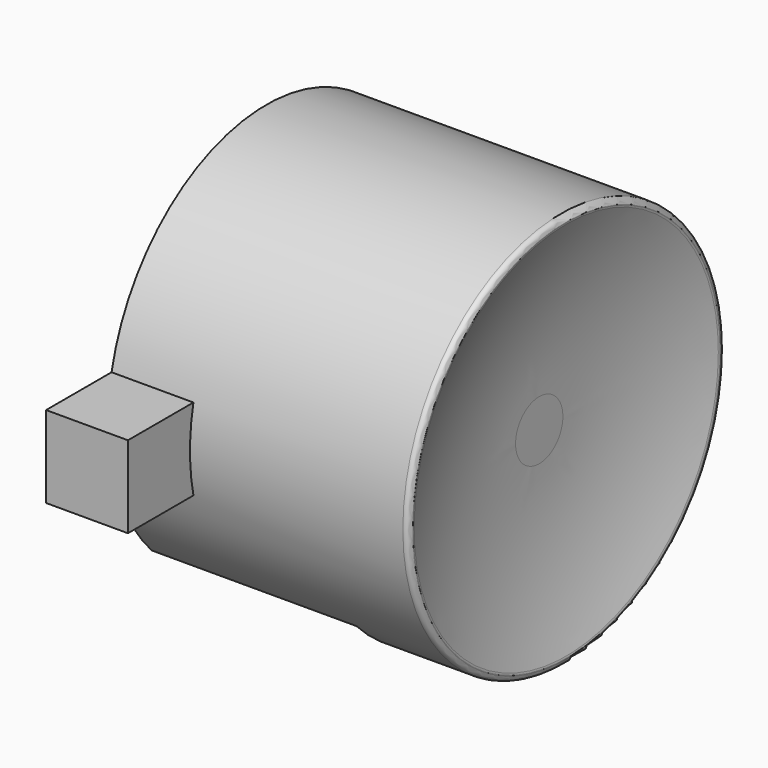
from build123d import *

# Parameters (mm, degrees)
F0_R     = 3.625
F1_DEPTH = 2.75
F3_DEPTH = 1.5
F4_R     = 3.5
F5_DEPTH = 0.5
F7_DEPTH = 3.75
F9_R     = 0.1


# Not quite as in the source:
# - a fillet or chamfer that OpenCascade refuses, or shapes differently, is made with other operations: its cross-section is extruded or revolved along the edge and cut away or added


with BuildPart() as f1:
    # F0 (on Right) → F1 (new body, symmetric)
    with BuildSketch(Plane.YZ):
        Circle(F0_R)
    extrude(amount=F1_DEPTH, both=True)

    # F2 (on face) → F3 (join)
    with BuildSketch(Plane(origin=(-2.75, 0, 0), x_dir=(0, -1, 0), z_dir=(-1, 0, 0))):
        with BuildLine():
            Line((3.5465652398, -0.75), (5.0465652398, -0.75))
            Line((5.0465652398, -0.75), (5.0465652398, 0.75))
            Line((5.0465652398, 0.75), (3.5465652398, 0.75))
            ThreePointArc((3.5465652398, 0.75), (3.625, 0), (3.5465652398, -0.75))
        make_face()
        with BuildLine():
            Line((-3.5465652398, 0.75), (-5.0465652398, 0.75))
            Line((-5.0465652398, 0.75), (-5.0465652398, -0.75))
            Line((-5.0465652398, -0.75), (-3.5465652398, -0.75))
            ThreePointArc((-3.5465652398, -0.75), (-3.625, 0), (-3.5465652398, 0.75))
        make_face()
    extrude(amount=-F3_DEPTH)

    # F4 (on face) → F5 (cut)
    with BuildSketch(Plane.YZ.offset(2.75)):
        Circle(F4_R)
    extrude(amount=-F5_DEPTH, mode=Mode.SUBTRACT)

    # F6 (on face) → F7 (cut)
    with BuildSketch(Plane(origin=(-2.75, 0, 0), x_dir=(0, -1, 0), z_dir=(-1, 0, 0))):
        with BuildLine():
            Line((2.625, -2.5), (-2.625, -2.5))
            ThreePointArc((-2.625, -2.5), (0, -3.625), (2.625, -2.5))
        make_face()
    extrude(amount=-F7_DEPTH, mode=Mode.SUBTRACT)

    # F8: fillet of radius 9 on 1 edges, made by hand

    # F8_s1 → F8_t2 (revolve)
    with BuildSketch(Plane.XY):
        with BuildLine():
            ThreePointArc((2.75, 3.5), (2.3758803254, 2.0419601084), (2.25, 0.5419601084))
            Line((2.25, 0.5419601084), (2.25, 3.5))
            Line((2.25, 3.5), (2.75, 3.5))
        make_face()
    revolve(axis=Axis((2.25, 0, 0), (1, 0, 0)))

    # F9
    f9_edges = [f1.edges().sort_by_distance(p)[0] for p in [
        (2.75, -3.5, 0),
        (2.75, -3.625, 0),
    ]]
    fillet(f9_edges, radius=F9_R)


solid = f1.part
